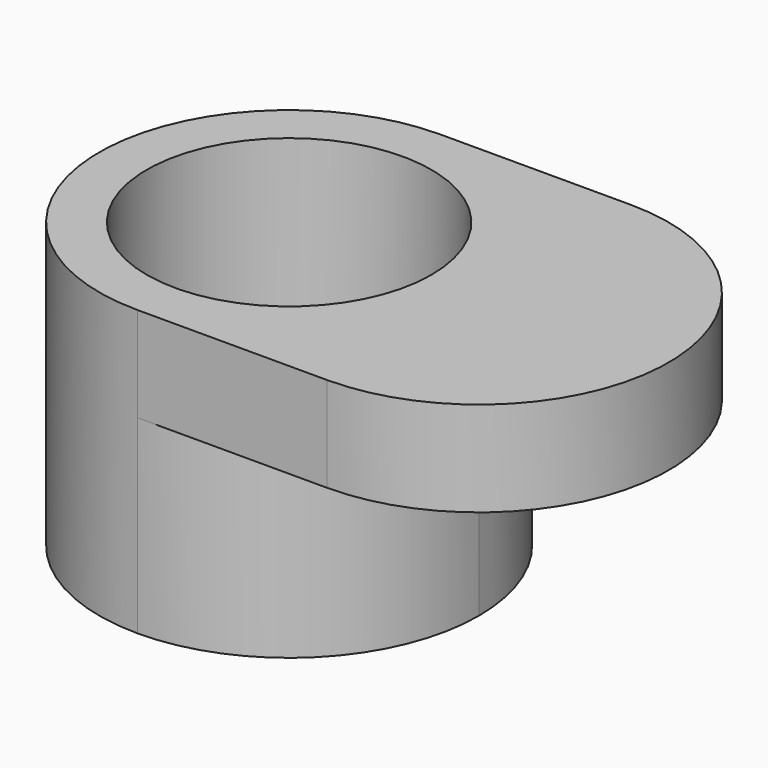
from build123d import *

# Parameters (mm, degrees)
F0_R     = 9.525
F1_DEPTH = 6.35
F2_R     = 9.525
F3_DEPTH = 12.7


# Not quite as in the source:
# - a length typed as a fraction of an inch, garbled in the dataset ("3 / 203.2 mm" for 3/8 in), is restored


with BuildPart() as f1:
    # F0 (on Top) → F1 (new body)
    with BuildSketch(Plane.XY):
        with BuildLine():
            Line((12.7, 12.7), (0, 12.7))
            ThreePointArc((0, 12.7), (-12.7, 0), (0, -12.7))
            Line((0, -12.7), (12.7, -12.7))
            ThreePointArc((12.7, -12.7), (25.4, 0), (12.7, 12.7))
        make_face()
        Circle(F0_R, mode=Mode.SUBTRACT)
    extrude(amount=F1_DEPTH)

    # F2 (on face) → F3 (join)
    with BuildSketch(Plane(origin=(0, 0, 0), x_dir=(1, 0, 0), z_dir=(0, 0, -1))):
        with BuildLine():
            ThreePointArc((0, -12.7), (8.9802561211, -8.9802561211), (12.7, 0))
            ThreePointArc((12.7, 0), (8.9802561211, 8.9802561211), (0, 12.7))
            ThreePointArc((0, 12.7), (-12.7, 0), (0, -12.7))
        make_face()
        Circle(F2_R, mode=Mode.SUBTRACT)
    extrude(amount=F3_DEPTH)


solid = f1.part
